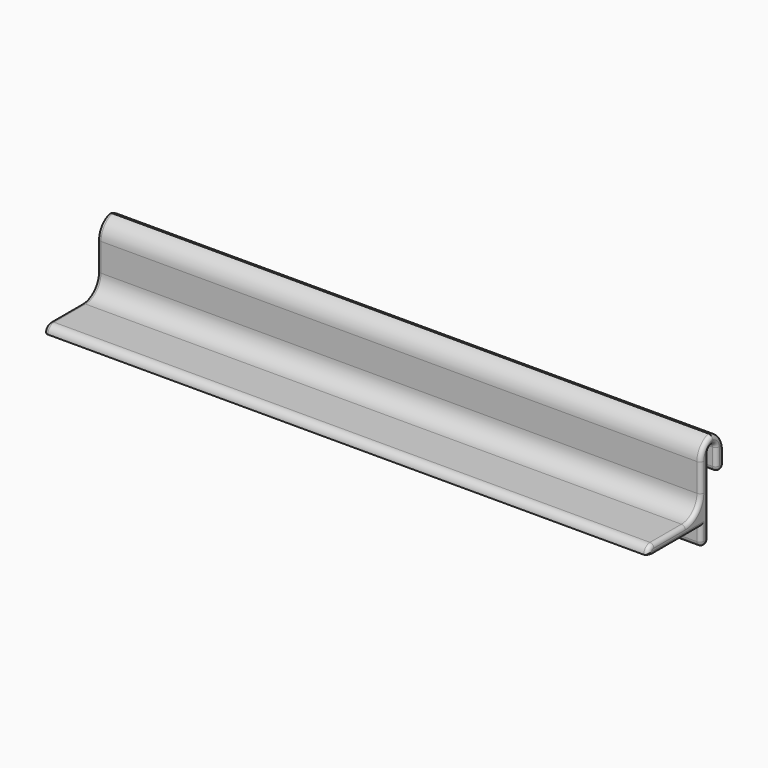
from build123d import *

# Parameters (mm, degrees)
F1_DEPTH     = 158.75
F2_R         = 2.032
F3_R         = 1.26999
F4_T1_DEPTH  = 169.8216033166
F5_T1_DEPTH  = 158.75
F5_T3_DEPTH  = 184.15
F6_T1_DEPTH  = 2e-05
F6_T3_DEPTH  = 4.44502
F6_T5_DEPTH  = 2e-05
F6_T7_DEPTH  = 19.81202
F6_T9_DEPTH  = 2e-05
F6_T11_DEPTH = 3.55601
F6_T13_DEPTH = 15.2481793367
F6_T15_DEPTH = 10.3505
F6_T17_DEPTH = 7.366
F6_T19_DEPTH = 3.17501
F6_T22_ANGLE = 90
F6_T24_ANGLE = 90
F6_T26_ANGLE = 90
F6_T28_ANGLE = 90
F6_T30_ANGLE = 90
F6_T32_ANGLE = 90
F6_T34_ANGLE = 54.4907710803
F6_T36_ANGLE = 161.6484946187
F6_T38_ANGLE = 89.9999999979
F6_T40_ANGLE = 104.1784803607
F6_T42_ANGLE = 104.1784803607
F6_T44_ANGLE = 90
F6_T46_ANGLE = 90
F6_T48_ANGLE = 90
F6_T50_ANGLE = 90
F6_T52_ANGLE = 90
F6_T54_ANGLE = 90
F6_T56_ANGLE = 54.4907710803
F6_T58_ANGLE = 161.6484946187
F6_T60_ANGLE = 89.9999999979
F6_T62_ANGLE = 104.1784803607
F6_T64_ANGLE = 104.1784803607
F6_T69_DEPTH = 6.09601
F6_T73_DEPTH = 17.7881793367
F6_T80_DEPTH = 6.09601
F6_T84_DEPTH = 17.7881793367


# Not quite as in the source:
# - a fillet or chamfer that OpenCascade refuses, or shapes differently, is made with other operations: its cross-section is extruded or revolved along the edge and cut away or added
# - a fillet or chamfer is up to 0.001 mm smaller than in the source, because OpenCascade refuses the exact size


with BuildPart() as f1:
    # F0 (on Right) → F1 (new body)
    with BuildSketch(Plane.YZ):
        Polygon((0, 17.526), (0, 0), (-17.4625, 0), (-17.4625, -2.54), (0, -2.54), (0, -7.366), (2.54, -7.366), (2.54, 14.986), (5.08, 14.986), (5.08, 8.001), (7.62, 8.001), (7.62, 17.526), align=None)
    extrude(amount=F1_DEPTH)

    # F2
    f2_edges = [f1.edges().sort_by_distance(p)[0] for p in [
        (79.375, -17.4625, 0),
    ]]
    fillet(f2_edges, radius=F2_R)

    # F3 (radius 1.27 in the source; OpenCascade refuses exactly that, so slightly less here)
    f3_edges = [f1.edges().sort_by_distance(p)[0] for p in [
        (79.375, 2.54, 14.986),
        (79.375, 5.08, 14.986),
        (79.375, 5.08, 8.001),
        (79.375, 7.62, 8.001),
        (79.375, 2.54, -7.366),
        (79.375, 0, -7.366),
    ]]
    fillet(f3_edges, radius=F3_R)

    # F4: fillet of radius 5.08 on 1 edges, made by hand

    # F4_s2 → F4_t1 (cut)
    with BuildSketch(Plane.YZ.offset(-5.5358016583)):
        with BuildLine():
            ThreePointArc((-17.4625, -2.032), (-16.3841018693, -2.4113715272), (-15.2481793367, -2.54))
            Line((-15.2481793367, -2.54), (-17.4625, -2.54))
            Line((-17.4625, -2.54), (-17.4625, -2.032))
        make_face()
    extrude(amount=F4_T1_DEPTH, mode=Mode.SUBTRACT)

    # F5: fillet of radius 5.08 on 3 edges, made by hand

    # F5_s2 → F5_t1 (join)
    with BuildSketch(Plane.YZ):
        with BuildLine():
            ThreePointArc((-5.08, 0), (-1.4878975516, 1.4878975516), (0, 5.08))
            Line((0, 5.08), (0, 0))
            Line((0, 0), (-5.08, 0))
        make_face()
    extrude(amount=F5_T1_DEPTH)

    # F5_s4 → F5_t3 (cut)
    with BuildSketch(Plane.YZ.offset(-12.7)):
        with BuildLine():
            ThreePointArc((0, 12.446), (1.4878975516, 16.0381024484), (5.08, 17.526))
            Line((5.08, 17.526), (0, 17.526))
            Line((0, 17.526), (0, 12.446))
        make_face()
        with BuildLine():
            ThreePointArc((2.54, 17.526), (6.1321024484, 16.0381024484), (7.62, 12.446))
            Line((7.62, 12.446), (7.62, 17.526))
            Line((7.62, 17.526), (2.54, 17.526))
        make_face()
    extrude(amount=F5_T3_DEPTH, mode=Mode.SUBTRACT)

    # F6: fillet of radius 1.016 on 42 edges, made by hand

    # F6_s2 → F6_t1 (cut)
    with BuildSketch(Plane.XZ.offset(-6.35001)):
        with BuildLine():
            ThreePointArc((157.734, 8.001), (158.4524204897, 8.2985795103), (158.75, 9.017))
            Line((158.75, 9.017), (158.75, 8.001))
            Line((158.75, 8.001), (157.734, 8.001))
        make_face()
        with BuildLine():
            ThreePointArc((0, 9.017), (0.2975795103, 8.2985795103), (1.016, 8.001))
            Line((1.016, 8.001), (0, 8.001))
            Line((0, 8.001), (0, 9.017))
        make_face()
    extrude(amount=F6_T1_DEPTH, mode=Mode.SUBTRACT)

    # F6_s4 → F6_t3 (cut)
    with BuildSketch(Plane.XY.offset(9.27099)):
        with BuildLine():
            ThreePointArc((157.734, 5.08), (158.4524204897, 5.3775795103), (158.75, 6.096))
            Line((158.75, 6.096), (158.75, 5.08))
            Line((158.75, 5.08), (157.734, 5.08))
        make_face()
        with BuildLine():
            ThreePointArc((0, 6.096), (0.2975795103, 5.3775795103), (1.016, 5.08))
            Line((1.016, 5.08), (0, 5.08))
            Line((0, 5.08), (0, 6.096))
        make_face()
    extrude(amount=F6_T3_DEPTH, mode=Mode.SUBTRACT)

    # F6_s6 → F6_t5 (cut)
    with BuildSketch(Plane.XZ.offset(-3.81001)):
        with BuildLine():
            ThreePointArc((157.734, 14.986), (158.4524204897, 15.2835795103), (158.75, 16.002))
            Line((158.75, 16.002), (158.75, 14.986))
            Line((158.75, 14.986), (157.734, 14.986))
        make_face()
        with BuildLine():
            ThreePointArc((0, 16.002), (0.2975795103, 15.2835795103), (1.016, 14.986))
            Line((1.016, 14.986), (0, 14.986))
            Line((0, 14.986), (0, 16.002))
        make_face()
    extrude(amount=F6_T5_DEPTH, mode=Mode.SUBTRACT)

    # F6_s8 → F6_t7 (cut)
    with BuildSketch(Plane.XY.offset(-6.09601)):
        with BuildLine():
            ThreePointArc((157.734, 2.54), (158.4524204897, 2.2424204897), (158.75, 1.524))
            Line((158.75, 1.524), (158.75, 2.54))
            Line((158.75, 2.54), (157.734, 2.54))
        make_face()
        with BuildLine():
            ThreePointArc((0, 1.524), (0.2975795103, 2.2424204897), (1.016, 2.54))
            Line((1.016, 2.54), (0, 2.54))
            Line((0, 2.54), (0, 1.524))
        make_face()
    extrude(amount=F6_T7_DEPTH, mode=Mode.SUBTRACT)

    # F6_s10 → F6_t9 (cut)
    with BuildSketch(Plane.XZ.offset(-1.27001)):
        with BuildLine():
            ThreePointArc((157.734, -7.366), (158.4524204897, -7.0684204897), (158.75, -6.35))
            Line((158.75, -6.35), (158.75, -7.366))
            Line((158.75, -7.366), (157.734, -7.366))
        make_face()
        with BuildLine():
            ThreePointArc((0, -6.35), (0.2975795103, -7.0684204897), (1.016, -7.366))
            Line((1.016, -7.366), (0, -7.366))
            Line((0, -7.366), (0, -6.35))
        make_face()
    extrude(amount=F6_T9_DEPTH, mode=Mode.SUBTRACT)

    # F6_s12 → F6_t11 (cut)
    with BuildSketch(Plane.XY.offset(-6.09601)):
        with BuildLine():
            ThreePointArc((157.734, 0), (158.4524204897, 0.2975795103), (158.75, 1.016))
            Line((158.75, 1.016), (158.75, 0))
            Line((158.75, 0), (157.734, 0))
        make_face()
        with BuildLine():
            ThreePointArc((0, 1.016), (0.2975795103, 0.2975795103), (1.016, 0))
            Line((1.016, 0), (0, 0))
            Line((0, 0), (0, 1.016))
        make_face()
    extrude(amount=F6_T11_DEPTH, mode=Mode.SUBTRACT)

    # F6_s14 → F6_t13 (cut)
    with BuildSketch(Plane.XZ):
        with BuildLine():
            ThreePointArc((157.734, -2.54), (158.4524204897, -2.2424204897), (158.75, -1.524))
            Line((158.75, -1.524), (158.75, -2.54))
            Line((158.75, -2.54), (157.734, -2.54))
        make_face()
        with BuildLine():
            ThreePointArc((0, -1.524), (0.2975795103, -2.2424204897), (1.016, -2.54))
            Line((1.016, -2.54), (0, -2.54))
            Line((0, -2.54), (0, -1.524))
        make_face()
    extrude(amount=F6_T13_DEPTH, mode=Mode.SUBTRACT)

    # F6_s16 → F6_t15 (cut)
    with BuildSketch(Plane.XZ.offset(5.08)):
        with BuildLine():
            ThreePointArc((157.734, 0), (158.4524204897, -0.2975795103), (158.75, -1.016))
            Line((158.75, -1.016), (158.75, 0))
            Line((158.75, 0), (157.734, 0))
        make_face()
        with BuildLine():
            ThreePointArc((0, -1.016), (0.2975795103, -0.2975795103), (1.016, 0))
            Line((1.016, 0), (0, 0))
            Line((0, 0), (0, -1.016))
        make_face()
    extrude(amount=F6_T15_DEPTH, mode=Mode.SUBTRACT)

    # F6_s18 → F6_t17 (cut)
    with BuildSketch(Plane.XY.offset(5.08)):
        with BuildLine():
            ThreePointArc((157.734, 0), (158.4524204897, 0.2975795103), (158.75, 1.016))
            Line((158.75, 1.016), (158.75, 0))
            Line((158.75, 0), (157.734, 0))
        make_face()
        with BuildLine():
            ThreePointArc((0, 1.016), (0.2975795103, 0.2975795103), (1.016, 0))
            Line((1.016, 0), (0, 0))
            Line((0, 0), (0, 1.016))
        make_face()
    extrude(amount=F6_T17_DEPTH, mode=Mode.SUBTRACT)

    # F6_s20 → F6_t19 (cut)
    with BuildSketch(Plane.XY.offset(9.27099)):
        with BuildLine():
            ThreePointArc((157.734, 7.62), (158.4524204897, 7.3224204897), (158.75, 6.604))
            Line((158.75, 6.604), (158.75, 7.62))
            Line((158.75, 7.62), (157.734, 7.62))
        make_face()
        with BuildLine():
            ThreePointArc((0, 6.604), (0.2975795103, 7.3224204897), (1.016, 7.62))
            Line((1.016, 7.62), (0, 7.62))
            Line((0, 7.62), (0, 6.604))
        make_face()
    extrude(amount=F6_T19_DEPTH, mode=Mode.SUBTRACT)

    # F6_s21 → F6_t22 (revolve, cut)
    with BuildSketch(Plane.XY.offset(9.27099)):
        with BuildLine():
            ThreePointArc((157.734, 7.62), (158.4524204897, 7.3224204897), (158.75, 6.604))
            Line((158.75, 6.604), (158.75, 7.62))
            Line((158.75, 7.62), (157.734, 7.62))
        make_face()
    revolve(axis=Axis((158.75, 6.35001, 9.27099), (-1, 0, 0)), revolution_arc=F6_T22_ANGLE, mode=Mode.SUBTRACT)

    # F6_s23 → F6_t24 (revolve, cut)
    with BuildSketch(Plane.XZ.offset(-6.34999)):
        with BuildLine():
            ThreePointArc((157.734, 8.001), (158.4524204897, 8.2985795103), (158.75, 9.017))
            Line((158.75, 9.017), (158.75, 8.001))
            Line((158.75, 8.001), (157.734, 8.001))
        make_face()
    revolve(axis=Axis((158.75, 6.34999, 9.27099), (-1, 0, 0)), revolution_arc=F6_T24_ANGLE, mode=Mode.SUBTRACT)

    # F6_s25 → F6_t26 (revolve, cut)
    with BuildSketch(Plane.XY.offset(13.71601)):
        with BuildLine():
            ThreePointArc((157.734, 5.08), (158.4524204897, 5.3775795103), (158.75, 6.096))
            Line((158.75, 6.096), (158.75, 5.08))
            Line((158.75, 5.08), (157.734, 5.08))
        make_face()
    revolve(axis=Axis((158.75, 3.81001, 13.71601), (1, 0, 0)), revolution_arc=F6_T26_ANGLE, mode=Mode.SUBTRACT)

    # F6_s27 → F6_t28 (revolve, cut)
    with BuildSketch(Plane.XY.offset(13.71601)):
        with BuildLine():
            ThreePointArc((157.734, 2.54), (158.4524204897, 2.2424204897), (158.75, 1.524))
            Line((158.75, 1.524), (158.75, 2.54))
            Line((158.75, 2.54), (157.734, 2.54))
        make_face()
    revolve(axis=Axis((158.75, 3.80999, 13.71601), (-1, 0, 0)), revolution_arc=F6_T28_ANGLE, mode=Mode.SUBTRACT)

    # F6_s29 → F6_t30 (revolve, cut)
    with BuildSketch(Plane.XZ.offset(-1.27001)):
        with BuildLine():
            ThreePointArc((157.734, -7.366), (158.4524204897, -7.0684204897), (158.75, -6.35))
            Line((158.75, -6.35), (158.75, -7.366))
            Line((158.75, -7.366), (157.734, -7.366))
        make_face()
    revolve(axis=Axis((158.75, 1.27001, -6.09601), (1, 0, 0)), revolution_arc=F6_T30_ANGLE, mode=Mode.SUBTRACT)

    # F6_s31 → F6_t32 (revolve, cut)
    with BuildSketch(Plane.XY.offset(-6.09601)):
        with BuildLine():
            ThreePointArc((157.734, 0), (158.4524204897, 0.2975795103), (158.75, 1.016))
            Line((158.75, 1.016), (158.75, 0))
            Line((158.75, 0), (157.734, 0))
        make_face()
    revolve(axis=Axis((158.75, 1.26999, -6.09601), (1, 0, 0)), revolution_arc=F6_T32_ANGLE, mode=Mode.SUBTRACT)

    # F6_s33 → F6_t34 (revolve, cut)
    with BuildSketch(Plane.XZ.offset(15.2481793371)):
        with BuildLine():
            ThreePointArc((157.734, -2.54), (158.4524204897, -2.2424204897), (158.75, -1.524))
            Line((158.75, -1.524), (158.75, -2.54))
            Line((158.75, -2.54), (157.734, -2.54))
        make_face()
    revolve(axis=Axis((158.75, -15.2481793371, 2.5399999982), (-1, 0, 0)), revolution_arc=F6_T34_ANGLE, mode=Mode.SUBTRACT)

    # F6_s35 → F6_t36 (revolve, cut)
    with BuildSketch(Plane.XZ.offset(15.4305)):
        with BuildLine():
            ThreePointArc((157.734, 0), (158.4524204897, -0.2975795103), (158.75, -1.016))
            Line((158.75, -1.016), (158.75, 0))
            Line((158.75, 0), (157.734, 0))
        make_face()
    revolve(axis=Axis((158.75, -15.4305, -2.032), (1, 0, 0)), revolution_arc=F6_T36_ANGLE, mode=Mode.SUBTRACT)

    # F6_s37 → F6_t38 (revolve, cut)
    with BuildSketch(Plane.XZ.offset(5.0800000001)):
        with BuildLine():
            ThreePointArc((157.734, 0), (158.4524204897, -0.2975795103), (158.75, -1.016))
            Line((158.75, -1.016), (158.75, 0))
            Line((158.75, 0), (157.734, 0))
        make_face()
    revolve(axis=Axis((158.75, -5.0800000001, 5.0800000001), (1, 0, 0)), revolution_arc=F6_T38_ANGLE, mode=Mode.SUBTRACT)

    # F6_s39 → F6_t40 (revolve, cut)
    with BuildSketch(Plane.XY.offset(12.4459999999)):
        with BuildLine():
            ThreePointArc((157.734, 0), (158.4524204897, 0.2975795103), (158.75, 1.016))
            Line((158.75, 1.016), (158.75, 0))
            Line((158.75, 0), (157.734, 0))
        make_face()
    revolve(axis=Axis((158.75, 5.0800000001, 12.4459999999), (-1, 0, 0)), revolution_arc=F6_T40_ANGLE, mode=Mode.SUBTRACT)

    # F6_s41 → F6_t42 (revolve, cut)
    with BuildSketch(Plane(origin=(0, 5.3433037504, 1.3499285295), x_dir=(1, 0, 0), z_dir=(0, -0.9695374162, -0.244943256))):
        with BuildLine():
            ThreePointArc((157.734, 16.5247068112), (158.4524204897, 16.2271273009), (158.75, 15.5087068112))
            Line((158.75, 15.5087068112), (158.75, 16.5247068112))
            Line((158.75, 16.5247068112), (157.734, 16.5247068112))
        make_face()
    revolve(axis=Axis((158.75, 2.5399999999, 12.4459999999), (-1, 0, 0)), revolution_arc=F6_T42_ANGLE, mode=Mode.SUBTRACT)

    # F6_s43 → F6_t44 (revolve, cut)
    with BuildSketch(Plane.XY.offset(9.27099)):
        with BuildLine():
            ThreePointArc((0, 6.604), (0.2975795103, 7.3224204897), (1.016, 7.62))
            Line((1.016, 7.62), (0, 7.62))
            Line((0, 7.62), (0, 6.604))
        make_face()
    revolve(axis=Axis((0, 6.35001, 9.27099), (-1, 0, 0)), revolution_arc=F6_T44_ANGLE, mode=Mode.SUBTRACT)

    # F6_s45 → F6_t46 (revolve, cut)
    with BuildSketch(Plane.XZ.offset(-6.34999)):
        with BuildLine():
            ThreePointArc((0, 9.017), (0.2975795103, 8.2985795103), (1.016, 8.001))
            Line((1.016, 8.001), (0, 8.001))
            Line((0, 8.001), (0, 9.017))
        make_face()
    revolve(axis=Axis((0, 6.34999, 9.27099), (-1, 0, 0)), revolution_arc=F6_T46_ANGLE, mode=Mode.SUBTRACT)

    # F6_s47 → F6_t48 (revolve, cut)
    with BuildSketch(Plane.XY.offset(13.71601)):
        with BuildLine():
            ThreePointArc((0, 6.096), (0.2975795103, 5.3775795103), (1.016, 5.08))
            Line((1.016, 5.08), (0, 5.08))
            Line((0, 5.08), (0, 6.096))
        make_face()
    revolve(axis=Axis((0, 3.81001, 13.71601), (1, 0, 0)), revolution_arc=F6_T48_ANGLE, mode=Mode.SUBTRACT)

    # F6_s49 → F6_t50 (revolve, cut)
    with BuildSketch(Plane.XY.offset(13.71601)):
        with BuildLine():
            ThreePointArc((0, 1.524), (0.2975795103, 2.2424204897), (1.016, 2.54))
            Line((1.016, 2.54), (0, 2.54))
            Line((0, 2.54), (0, 1.524))
        make_face()
    revolve(axis=Axis((0, 3.80999, 13.71601), (-1, 0, 0)), revolution_arc=F6_T50_ANGLE, mode=Mode.SUBTRACT)

    # F6_s51 → F6_t52 (revolve, cut)
    with BuildSketch(Plane.XZ.offset(-1.27001)):
        with BuildLine():
            ThreePointArc((0, -6.35), (0.2975795103, -7.0684204897), (1.016, -7.366))
            Line((1.016, -7.366), (0, -7.366))
            Line((0, -7.366), (0, -6.35))
        make_face()
    revolve(axis=Axis((0, 1.27001, -6.09601), (1, 0, 0)), revolution_arc=F6_T52_ANGLE, mode=Mode.SUBTRACT)

    # F6_s53 → F6_t54 (revolve, cut)
    with BuildSketch(Plane.XY.offset(-6.09601)):
        with BuildLine():
            ThreePointArc((0, 1.016), (0.2975795103, 0.2975795103), (1.016, 0))
            Line((1.016, 0), (0, 0))
            Line((0, 0), (0, 1.016))
        make_face()
    revolve(axis=Axis((0, 1.26999, -6.09601), (1, 0, 0)), revolution_arc=F6_T54_ANGLE, mode=Mode.SUBTRACT)

    # F6_s55 → F6_t56 (revolve, cut)
    with BuildSketch(Plane.XZ.offset(15.2481793371)):
        with BuildLine():
            ThreePointArc((0, -1.524), (0.2975795103, -2.2424204897), (1.016, -2.54))
            Line((1.016, -2.54), (0, -2.54))
            Line((0, -2.54), (0, -1.524))
        make_face()
    revolve(axis=Axis((0, -15.2481793371, 2.5399999982), (-1, 0, 0)), revolution_arc=F6_T56_ANGLE, mode=Mode.SUBTRACT)

    # F6_s57 → F6_t58 (revolve, cut)
    with BuildSketch(Plane.XZ.offset(15.4305)):
        with BuildLine():
            ThreePointArc((0, -1.016), (0.2975795103, -0.2975795103), (1.016, 0))
            Line((1.016, 0), (0, 0))
            Line((0, 0), (0, -1.016))
        make_face()
    revolve(axis=Axis((0, -15.4305, -2.032), (1, 0, 0)), revolution_arc=F6_T58_ANGLE, mode=Mode.SUBTRACT)

    # F6_s59 → F6_t60 (revolve, cut)
    with BuildSketch(Plane.XZ.offset(5.0800000001)):
        with BuildLine():
            ThreePointArc((0, -1.016), (0.2975795103, -0.2975795103), (1.016, 0))
            Line((1.016, 0), (0, 0))
            Line((0, 0), (0, -1.016))
        make_face()
    revolve(axis=Axis((0, -5.0800000001, 5.0800000001), (1, 0, 0)), revolution_arc=F6_T60_ANGLE, mode=Mode.SUBTRACT)

    # F6_s61 → F6_t62 (revolve, cut)
    with BuildSketch(Plane.XY.offset(12.4459999999)):
        with BuildLine():
            ThreePointArc((0, 1.016), (0.2975795103, 0.2975795103), (1.016, 0))
            Line((1.016, 0), (0, 0))
            Line((0, 0), (0, 1.016))
        make_face()
    revolve(axis=Axis((0, 5.0800000001, 12.4459999999), (-1, 0, 0)), revolution_arc=F6_T62_ANGLE, mode=Mode.SUBTRACT)

    # F6_s63 → F6_t64 (revolve, cut)
    with BuildSketch(Plane(origin=(0, 5.3433037504, 1.3499285295), x_dir=(1, 0, 0), z_dir=(0, -0.9695374162, -0.244943256))):
        with BuildLine():
            ThreePointArc((0, 15.5087068112), (0.2975795103, 16.2271273009), (1.016, 16.5247068112))
            Line((1.016, 16.5247068112), (0, 16.5247068112))
            Line((0, 16.5247068112), (0, 15.5087068112))
        make_face()
    revolve(axis=Axis((0, 2.5399999999, 12.4459999999), (-1, 0, 0)), revolution_arc=F6_T64_ANGLE, mode=Mode.SUBTRACT)


with BuildPart() as f6_tool67:
    # F6_s68 → F6_t69 (new body)
    with BuildSketch(Plane.XY):
        with BuildLine():
            ThreePointArc((157.734, 0), (158.4524204897, 0.2975795103), (158.75, 1.016))
            Line((158.75, 1.016), (158.75, 0))
            Line((158.75, 0), (157.734, 0))
        make_face()
    extrude(amount=-F6_T69_DEPTH)

    split(bisect_by=Plane.XY.offset(-2.54), keep=Keep.TOP)


with BuildPart() as f6_tool71:
    # F6_s72 → F6_t73 (new body)
    with BuildSketch(Plane.XZ.offset(15.2481793367)):
        with BuildLine():
            ThreePointArc((157.734, -2.54), (158.4524204897, -2.2424204897), (158.75, -1.524))
            Line((158.75, -1.524), (158.75, -2.54))
            Line((158.75, -2.54), (157.734, -2.54))
        make_face()
    extrude(amount=-F6_T73_DEPTH)

    split(bisect_by=Plane.XZ, keep=Keep.BOTTOM)


with BuildPart() as f6_tool67_1:
    add(f6_tool67.part)

    # F6_t75: intersect F6_tool71
    add(f6_tool71.part, mode=Mode.INTERSECT)


with BuildPart() as f1_1:
    add(f1.part)

    # F6_t65: cut F6_tool67
    add(f6_tool67_1.part, mode=Mode.SUBTRACT)


with BuildPart() as f6_tool78:
    # F6_s79 → F6_t80 (new body)
    with BuildSketch(Plane.XY):
        with BuildLine():
            ThreePointArc((0, 1.016), (0.2975795103, 0.2975795103), (1.016, 0))
            Line((1.016, 0), (0, 0))
            Line((0, 0), (0, 1.016))
        make_face()
    extrude(amount=-F6_T80_DEPTH)

    split(bisect_by=Plane.XY.offset(-2.54), keep=Keep.TOP)


with BuildPart() as f6_tool82:
    # F6_s83 → F6_t84 (new body)
    with BuildSketch(Plane.XZ.offset(15.2481793367)):
        with BuildLine():
            ThreePointArc((0, -1.524), (0.2975795103, -2.2424204897), (1.016, -2.54))
            Line((1.016, -2.54), (0, -2.54))
            Line((0, -2.54), (0, -1.524))
        make_face()
    extrude(amount=-F6_T84_DEPTH)

    split(bisect_by=Plane.XZ, keep=Keep.BOTTOM)


with BuildPart() as f6_tool78_1:
    add(f6_tool78.part)

    # F6_t86: intersect F6_tool82
    add(f6_tool82.part, mode=Mode.INTERSECT)


with BuildPart() as f1_2:
    add(f1_1.part)

    # F6_t76: cut F6_tool78
    add(f6_tool78_1.part, mode=Mode.SUBTRACT)


solid = f1_2.part
